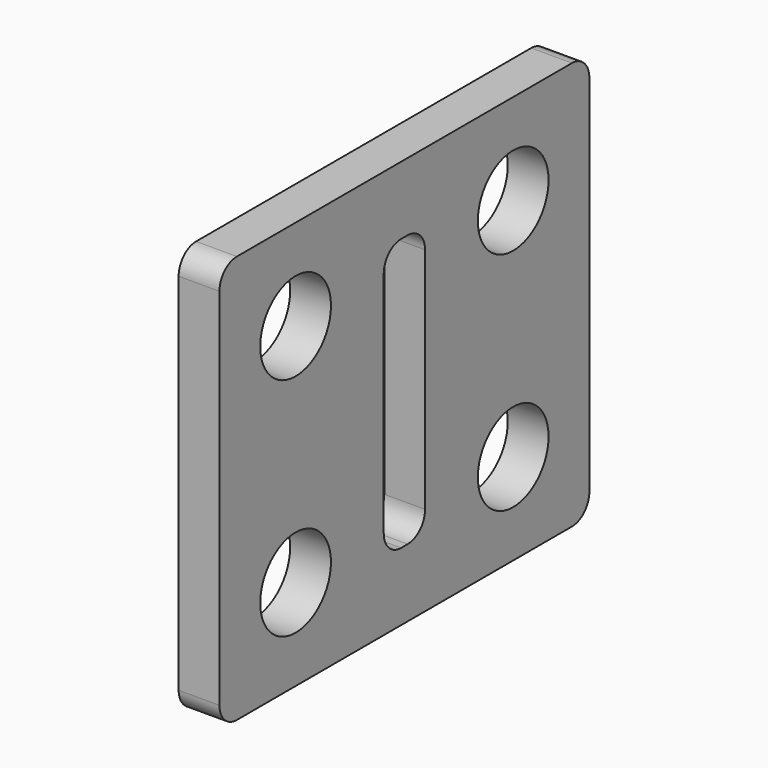
from build123d import *

# Parameters (mm, degrees)
F0_W           = 34
F0_H           = 30
F0_W_2         = 3.8
F0_H_2         = 20
F1_DEPTH       = 3
F2_R           = 1.6
F3_D           = 3.3
F3_CBORE_D     = 6.5
F3_CBORE_DEPTH = 3


# Not quite as in the source:
# - a feature names something its author has since deleted; it is built from what else it names


with BuildPart() as f1:
    # F0 (on Right) → F1 (new body)
    with BuildSketch(Plane.YZ):
        Rectangle(F0_W, F0_H)
        Rectangle(F0_W_2, F0_H_2, mode=Mode.SUBTRACT)
    extrude(amount=F1_DEPTH)

    # F2
    f2_edges = [f1.edges().sort_by_distance(p)[0] for p in [
        (1.5, -1.9, 10),
        (1.5, 1.9, 10),
        (1.5, -1.9, -10),
        (1.5, 1.9, -10),
        (1.5, -17, 15),
        (1.5, 17, 15),
        (1.5, 17, -15),
        (1.5, -17, -15),
    ]]
    fillet(f2_edges, radius=F2_R)

    # F3 (through all)
    with Locations(Plane(origin=(0, 0, 0), x_dir=(0, 1, 0), z_dir=(-1, 0, 0))):
        with Locations((10, -8.3), (-10, -8.3), (-10, 8.3), (10, 8.3)):
            CounterBoreHole(F3_D / 2, F3_CBORE_D / 2, F3_CBORE_DEPTH)


solid = f1.part
